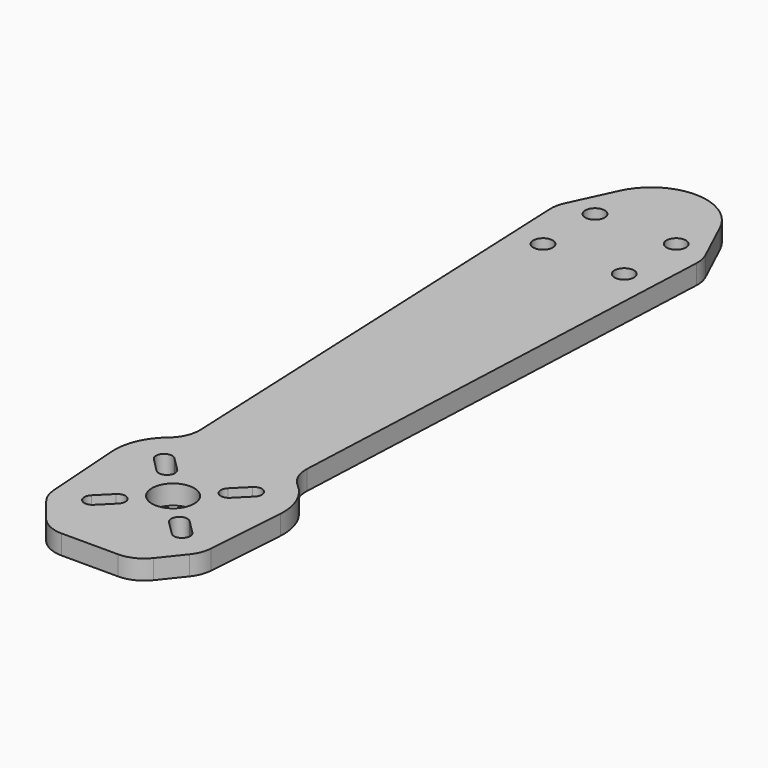
from build123d import *

# Parameters (mm, degrees)
F0_R     = 3.25
F0_R_2   = 1.5
F1_DEPTH = 3


# Not quite as in the source:
# - ends of sketch curves that miss each other by under 0.0002 mm in the source are joined


with BuildPart() as f1:
    # F0 (on Top) → F1 (new body)
    with BuildSketch(Plane.XY):
        with BuildLine():
            Line((8.1815379971, -26.6895870666), (11.2823570029, 44.3308440666))
            ThreePointArc((11.2823570029, 44.3308440666), (11.1910423827, 45.524392707), (10.8186548512, 46.6620324888))
            Line((10.8186548512, 46.6620324888), (7.703615805, 53.3422554181))
            ThreePointArc((7.703615805, 53.3422554181), (0, 58.25), (-7.703616047, 53.342255531))
            Line((-7.703616047, 53.342255531), (-10.8186551692, 46.6620326371))
            ThreePointArc((-10.8186551692, 46.6620326371), (-11.1910423827, 45.524392707), (-11.2823571079, 44.330844062))
            Line((-11.2823571079, 44.330844062), (-8.1815379971, -26.6895870666))
            ThreePointArc((-8.1815379971, -26.6895870666), (-8.6003047113, -28.9216063136), (-9.9631570958, -30.7381714698))
            ThreePointArc((-9.9631570958, -30.7381714698), (-12.3241540982, -33.9284623067), (-12.9792944589, -37.8429295738))
            Line((-12.9792944589, -37.8429295738), (-12.1222819893, -50.0987821525))
            ThreePointArc((-12.1222819893, -50.0987821525), (-11.7945005071, -51.5621897781), (-11.0475021701, -52.8625726982))
            Line((-11.0475021701, -52.8625726982), (-8.263477213, -56.3625727323))
            ThreePointArc((-8.263477213, -56.3625727323), (-6.5226625661, -57.753491062), (-4.350436, -58.25))
            Line((-4.350436, -58.25), (4.350436, -58.25))
            ThreePointArc((4.350436, -58.25), (6.5226625661, -57.753491062), (8.2634771701, -56.3625726982))
            Line((8.2634771701, -56.3625726982), (11.047502213, -52.8625727323))
            ThreePointArc((11.047502213, -52.8625727323), (11.7945005071, -51.5621897781), (12.1222812699, -50.0987821022))
            Line((12.1222812699, -50.0987821022), (12.9792940319, -37.8429295439))
            ThreePointArc((12.9792940319, -37.8429295439), (12.3241540982, -33.9284623067), (9.9631572372, -30.7381713013))
            ThreePointArc((9.9631572372, -30.7381713013), (8.6003047113, -28.9216063136), (8.1815379971, -26.6895870666))
        make_face()
        with BuildLine():
            Line((-3.8890875, -47.9068545), (-6.0104075, -50.0281745))
            ThreePointArc((-6.0104075235, -50.0281744765), (-7.7781744765, -50.0281744765), (-7.7781744765, -48.2604075235))
            Line((-7.7781745, -48.2604075), (-5.6568545, -46.1390875))
            ThreePointArc((-5.6568544765, -46.1390875235), (-3.8890875235, -46.1390875235), (-3.8890875235, -47.9068544765))
        make_face(mode=Mode.SUBTRACT)
        with BuildLine():
            ThreePointArc((-7.7781744765, -36.2395924765), (-7.7781744765, -34.4718255235), (-6.0104075235, -34.4718255235))
            Line((-6.0104075, -34.4718255), (-3.8890875, -36.5931455))
            ThreePointArc((-3.8890875235, -36.5931455235), (-3.8890875235, -38.3609124765), (-5.6568544765, -38.3609124765))
            Line((-5.6568545, -38.3609125), (-7.7781745, -36.2395925))
        make_face(mode=Mode.SUBTRACT)
        with Locations((0, -42.25)):
            Circle(F0_R, mode=Mode.SUBTRACT)
        with BuildLine():
            ThreePointArc((3.8890875235, -47.9068544765), (3.8890875235, -46.1390875235), (5.6568544765, -46.1390875235))
            Line((5.6568545, -46.1390875), (7.7781745, -48.2604075))
            ThreePointArc((7.7781744765, -48.2604075235), (7.7781744765, -50.0281744765), (6.0104075235, -50.0281744765))
            Line((6.0104075, -50.0281745), (3.8890875, -47.9068545))
        make_face(mode=Mode.SUBTRACT)
        with BuildLine():
            ThreePointArc((5.6568544765, -38.3609124765), (3.8890875235, -38.3609124765), (3.8890875235, -36.5931455235))
            Line((3.8890875, -36.5931455), (6.0104075, -34.4718255))
            ThreePointArc((6.0104075235, -34.4718255235), (7.7781744765, -34.4718255235), (7.7781744765, -36.2395924765))
            Line((7.7781745, -36.2395925), (5.6568545, -38.3609125))
        make_face(mode=Mode.SUBTRACT)
        with Locations((-6.25, 36.75)):
            Circle(F0_R_2, mode=Mode.SUBTRACT)
        with Locations((-6.25, 46.75)):
            Circle(F0_R_2, mode=Mode.SUBTRACT)
        with Locations((6.25, 36.75)):
            Circle(F0_R_2, mode=Mode.SUBTRACT)
        with Locations((6.25, 46.75)):
            Circle(F0_R_2, mode=Mode.SUBTRACT)
    extrude(amount=F1_DEPTH)


solid = f1.part
